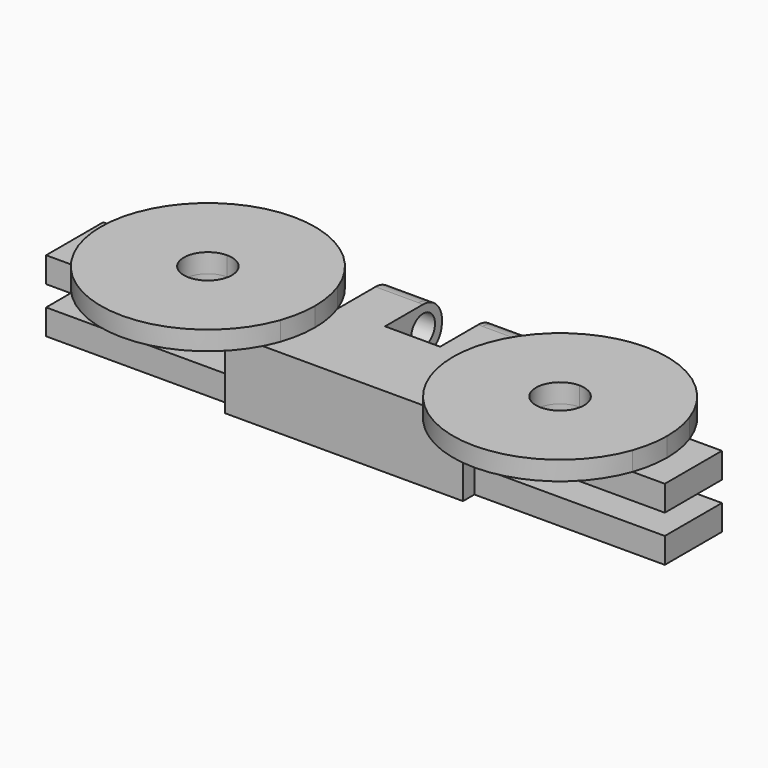
from build123d import *

# Parameters (mm, degrees)
F0_W         = 330.2
F0_H         = 38.1
F1_DEPTH     = 38.1
F2_W         = 19.05
F2_H         = 10.922
F3_DEPTH     = 101.6
F4_W         = 19.05
F4_H         = 10.922
F5_DEPTH     = 101.6
F7_DEPTH     = 22.86
F8_DEPTH     = 10.16
F10_DEPTH    = 7.62
F11_W        = 25.4
F11_H        = 13.589
F11_H_2      = 10.922
F12_DEPTH    = 38.1
F13_T1_DEPTH = 88.9
F13_T3_DEPTH = 88.9
F14_R        = 12.7
F16_DEPTH    = 101.6


# Not quite as in the source:
# - a fillet or chamfer that OpenCascade refuses, or shapes differently, is made with other operations: its cross-section is extruded or revolved along the edge and cut away or added
# - after a boolean that leaves OpenCascade's solid faulty, fix() repairs it
# - a feature names something its author has since deleted; it is built from what else it names


with BuildPart() as f1:
    # F0 (on Top) → F1 (new body)
    with BuildSketch(Plane.XY):
        Rectangle(F0_W, F0_H)
    extrude(amount=F1_DEPTH)

    # F2 (on face) → F3 (cut)
    with BuildSketch(Plane(origin=(-165.1, 0, 0), x_dir=(0, -1, 0), z_dir=(-1, 0, 0))):
        with Locations((9.525, 19.05)):
            Rectangle(F2_W, F2_H)
        with Locations((-9.525, 19.05)):
            Rectangle(F2_W, F2_H)
    extrude(amount=-F3_DEPTH, mode=Mode.SUBTRACT)

    # F4 (on face) → F5 (cut)
    with BuildSketch(Plane.YZ.offset(165.1)):
        with Locations((-9.525, 19.05)):
            Rectangle(F4_W, F4_H)
        with Locations((9.525, 19.05)):
            Rectangle(F4_W, F4_H)
    extrude(amount=-F5_DEPTH, mode=Mode.SUBTRACT)

    # F6 (on face) → F7 (cut)
    with BuildSketch(Plane.XY.offset(38.1)):
        with BuildLine():
            Line((-93.98, 12.827), (-93.98, -12.827))
            ThreePointArc((-93.98, -12.827), (-84.9099413177, -9.0700586823), (-81.153, 0))
            ThreePointArc((-81.153, 0), (-84.9099413177, 9.0700586823), (-93.98, 12.827))
        make_face()
        with BuildLine():
            ThreePointArc((-93.98, 12.827), (-106.807, 0), (-93.98, -12.827))
            Line((-93.98, -12.827), (-93.98, 12.827))
        make_face()
        with BuildLine():
            ThreePointArc((93.98, 12.827), (81.153, 0), (93.98, -12.827))
            Line((93.98, -12.827), (93.98, 12.827))
        make_face()
        with BuildLine():
            Line((93.98, 12.827), (93.98, -12.827))
            ThreePointArc((93.98, -12.827), (103.0500586823, -9.0700586823), (106.807, 0))
            ThreePointArc((106.807, 0), (103.0500586823, 9.0700586823), (93.98, 12.827))
        make_face()
    extrude(amount=-F7_DEPTH, mode=Mode.SUBTRACT)

    # F6 (on face) → F8 (join)
    with BuildSketch(Plane.XY.offset(38.1)):
        with BuildLine():
            ThreePointArc((110.7805208253, 19.05), (93.98, 25.4), (77.1794791747, 19.05))
            Line((77.1794791747, 19.05), (93.98, 19.05))
            Line((93.98, 19.05), (110.7805208253, 19.05))
        make_face()
        with BuildLine():
            Line((110.7805208253, -19.05), (147.8615367264, -19.05))
            ThreePointArc((147.8615367264, -19.05), (150.3069576842, -9.6641780842), (151.13, 0))
            ThreePointArc((151.13, 0), (150.3069576842, 9.6641780842), (147.8615367264, 19.05))
            Line((147.8615367264, 19.05), (110.7805208253, 19.05))
            ThreePointArc((110.7805208253, 19.05), (117.1305208253, 10.4505208253), (119.38, 0))
            ThreePointArc((119.38, 0), (117.1305208253, -10.4505208253), (110.7805208253, -19.05))
        make_face()
        with BuildLine():
            ThreePointArc((147.8615367264, 19.05), (93.98, 57.15), (40.0984632736, 19.05))
            Line((40.0984632736, 19.05), (77.1794791747, 19.05))
            ThreePointArc((77.1794791747, 19.05), (93.98, 25.4), (110.7805208253, 19.05))
            Line((110.7805208253, 19.05), (147.8615367264, 19.05))
        make_face()
        with BuildLine():
            ThreePointArc((77.1794791747, 19.05), (68.58, 0), (77.1794791747, -19.05))
            Line((77.1794791747, -19.05), (93.98, -19.05))
            Line((93.98, -19.05), (93.98, -12.827))
            ThreePointArc((93.98, -12.827), (81.153, 0), (93.98, 12.827))
            Line((93.98, 12.827), (93.98, 19.05))
            Line((93.98, 19.05), (77.1794791747, 19.05))
        make_face()
        with BuildLine():
            Line((93.98, -19.05), (110.7805208253, -19.05))
            ThreePointArc((110.7805208253, -19.05), (117.1305208253, -10.4505208253), (119.38, 0))
            ThreePointArc((119.38, 0), (117.1305208253, 10.4505208253), (110.7805208253, 19.05))
            Line((110.7805208253, 19.05), (93.98, 19.05))
            Line((93.98, 19.05), (93.98, 12.827))
            ThreePointArc((93.98, 12.827), (103.0500586823, 9.0700586823), (106.807, 0))
            ThreePointArc((106.807, 0), (103.0500586823, -9.0700586823), (93.98, -12.827))
            Line((93.98, -12.827), (93.98, -19.05))
        make_face()
        with BuildLine():
            ThreePointArc((40.0984632736, 19.05), (36.83, 0), (40.0984632736, -19.05))
            Line((40.0984632736, -19.05), (77.1794791747, -19.05))
            ThreePointArc((77.1794791747, -19.05), (68.58, 0), (77.1794791747, 19.05))
            Line((77.1794791747, 19.05), (40.0984632736, 19.05))
        make_face()
        with BuildLine():
            Line((77.1794791747, -19.05), (40.0984632736, -19.05))
            ThreePointArc((40.0984632736, -19.05), (93.98, -57.15), (147.8615367264, -19.05))
            Line((147.8615367264, -19.05), (110.7805208253, -19.05))
            ThreePointArc((110.7805208253, -19.05), (93.98, -25.4), (77.1794791747, -19.05))
        make_face()
        with BuildLine():
            Line((93.98, -19.05), (77.1794791747, -19.05))
            ThreePointArc((77.1794791747, -19.05), (93.98, -25.4), (110.7805208253, -19.05))
            Line((110.7805208253, -19.05), (93.98, -19.05))
        make_face()
        with BuildLine():
            Line((-93.98, -12.827), (-93.98, -19.05))
            Line((-93.98, -19.05), (-40.0984632736, -19.05))
            ThreePointArc((-40.0984632736, -19.05), (-37.6530423158, -9.6641780842), (-36.83, 0))
            ThreePointArc((-36.83, 0), (-37.6530423158, 9.6641780842), (-40.0984632736, 19.05))
            Line((-40.0984632736, 19.05), (-93.98, 19.05))
            Line((-93.98, 19.05), (-93.98, 12.827))
            ThreePointArc((-93.98, 12.827), (-84.9099413177, 9.0700586823), (-81.153, 0))
            ThreePointArc((-81.153, 0), (-84.9099413177, -9.0700586823), (-93.98, -12.827))
        make_face()
        with BuildLine():
            Line((-147.8615367264, -19.05), (-93.98, -19.05))
            Line((-93.98, -19.05), (-93.98, -12.827))
            ThreePointArc((-93.98, -12.827), (-106.807, 0), (-93.98, 12.827))
            Line((-93.98, 12.827), (-93.98, 19.05))
            Line((-93.98, 19.05), (-147.8615367264, 19.05))
            ThreePointArc((-147.8615367264, 19.05), (-151.13, 0), (-147.8615367264, -19.05))
        make_face()
        with BuildLine():
            Line((-40.0984632736, -19.05), (-93.98, -19.05))
            Line((-93.98, -19.05), (-147.8615367264, -19.05))
            ThreePointArc((-147.8615367264, -19.05), (-93.98, -57.15), (-40.0984632736, -19.05))
        make_face()
        with BuildLine():
            ThreePointArc((-40.0984632736, 19.05), (-93.98, 57.15), (-147.8615367264, 19.05))
            Line((-147.8615367264, 19.05), (-93.98, 19.05))
            Line((-93.98, 19.05), (-40.0984632736, 19.05))
        make_face()
    extrude(amount=F8_DEPTH)

    # F9 (on face) → F10 (join)
    with BuildSketch(Plane.XZ.offset(19.05)):
        Polygon((0, 0), (0, 38.1), (-40.0984632736, 38.1), (-63.5, 38.1), (-63.5, 30.861), (-63.5, 24.511), (-63.5, 19.939), (-63.5, 13.589), (-63.5, 0), align=None)
        Polygon((63.5, 30.861), (63.5, 38.1), (40.0984632736, 38.1), (13.5538854515, 38.1), (0, 38.1), (0, 0), (63.5, 0), (63.5, 13.589), (63.5, 19.939), (63.5, 24.511), align=None)
    extrude(amount=F10_DEPTH)

    add(f1.part.fix(), mode=Mode.REPLACE)

    # F11 (on face) → F12 (join)
    with BuildSketch(Plane(origin=(0, 19.05, 0), x_dir=(-1, 0, 0), z_dir=(0, 1, 0))):
        with Locations((-27.3984632736, 31.3055)):
            Rectangle(F11_W, F11_H)
        with Locations((-27.3984632736, 19.05)):
            Rectangle(F11_W, F11_H_2)
        with Locations((27.3984632736, 19.05)):
            Rectangle(F11_W, F11_H_2)
        with Locations((27.3984632736, 31.3055)):
            Rectangle(F11_W, F11_H)
    extrude(amount=F12_DEPTH)

    # F13: fillet of radius 12.7 on 2 edges, made by hand

    # F13_s2 → F13_t1 (cut)
    with BuildSketch(Plane.YZ.offset(-71.8484632736)):
        with BuildLine():
            add(Edge.make_bspline(
                [(44.45, 13.589), (57.15, 13.589), (57.15, 26.289)],
                knots=[0, 0, 0, 1, 1, 1], degree=2, weights=[1, 1, 1]))
            Line((57.15, 26.289), (57.15, 13.589))
            Line((57.15, 13.589), (44.45, 13.589))
        make_face()
    extrude(amount=F13_T1_DEPTH, mode=Mode.SUBTRACT)

    # F13_s4 → F13_t3 (cut)
    with BuildSketch(Plane.YZ.offset(-17.0515367264)):
        with BuildLine():
            add(Edge.make_bspline(
                [(44.45, 13.589), (57.15, 13.589), (57.15, 26.289)],
                knots=[0, 0, 0, 1, 1, 1], degree=2, weights=[1, 1, 1]))
            Line((57.15, 26.289), (57.15, 13.589))
            Line((57.15, 13.589), (44.45, 13.589))
        make_face()
    extrude(amount=F13_T3_DEPTH, mode=Mode.SUBTRACT)

    # F14
    f14_edges = [f1.edges().sort_by_distance(p)[0] for p in [
        (27.398463, 57.15, 38.1),
        (-27.398463, 57.15, 38.1),
    ]]
    fillet(f14_edges, radius=F14_R)

    # F15 (on face) → F16 (cut)
    with BuildSketch(Plane(origin=(-40.0984632736, 0, 0), x_dir=(0, -1, 0), z_dir=(-1, 0, 0))):
        with BuildLine():
            ThreePointArc((-52.3875, 25.8445), (-44.45, 17.907), (-36.5125, 25.8445))
            Line((-36.5125, 25.8445), (-52.3875, 25.8445))
        make_face()
        with BuildLine():
            Line((-52.3875, 25.8445), (-36.5125, 25.8445))
            ThreePointArc((-36.5125, 25.8445), (-44.45, 33.782), (-52.3875, 25.8445))
        make_face()
    extrude(amount=-F16_DEPTH, mode=Mode.SUBTRACT)


solid = f1.part
